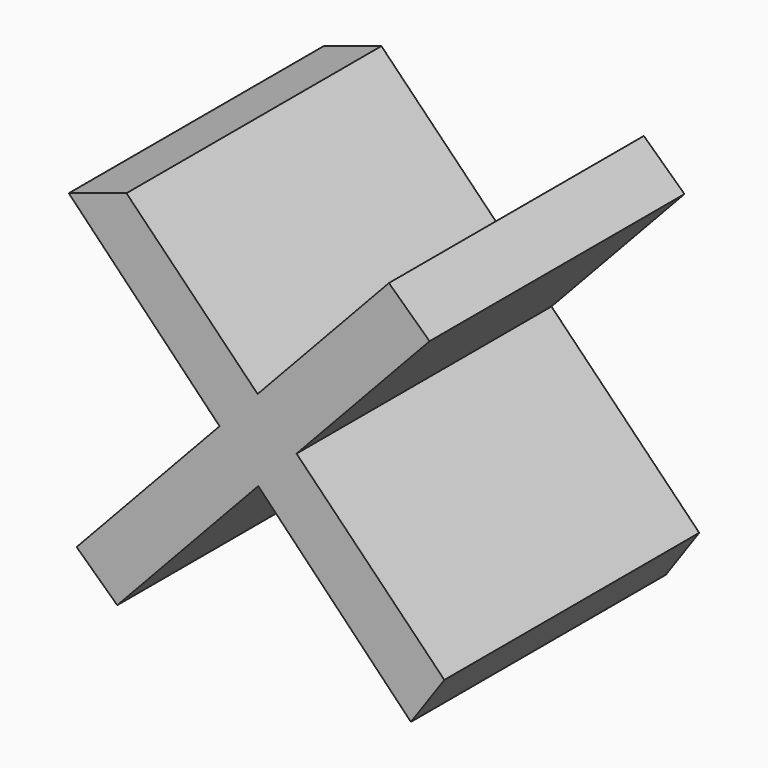
from build123d import *

# Parameters (mm, degrees)
F1_DEPTH = 53


# Not quite as in the source:
# - a feature names something its author has since deleted; it is built from what else it names


with BuildPart() as f1:
    # F0 (on Front) → F1 (new body)
    with BuildSketch(Plane.XZ):
        Polygon((-30.7423530247, 26.6767482577), (-5.6632759116, 0.7168226163), (0.6696432283, 7.4890868759), (-21.1426665217, 29.8010575561), align=None)
        Polygon((7.143901395, 0.8665209922), (29.2684723572, 24.5259800626), (22.5106922376, 30.8453547093), (0.6696432283, 7.4890868759), align=None)
        Polygon((0.7734024336, -5.9459301822), (26.1681957986, -32.2326609282), (31.7237185496, -24.2763531905), (7.143901395, 0.8665209922), align=None)
        Polygon((-5.6632759116, 0.7168226163), (0.7734024336, -5.9459301822), (7.143901395, 0.8665209922), (0.6696432283, 7.4890868759), align=None)
        Polygon((-29.4360663926, -24.7052009039), (-22.678286273, -31.0245755505), (0.7734024336, -5.9459301822), (-5.6632759116, 0.7168226163), align=None)
    extrude(amount=-F1_DEPTH)


solid = f1.part
